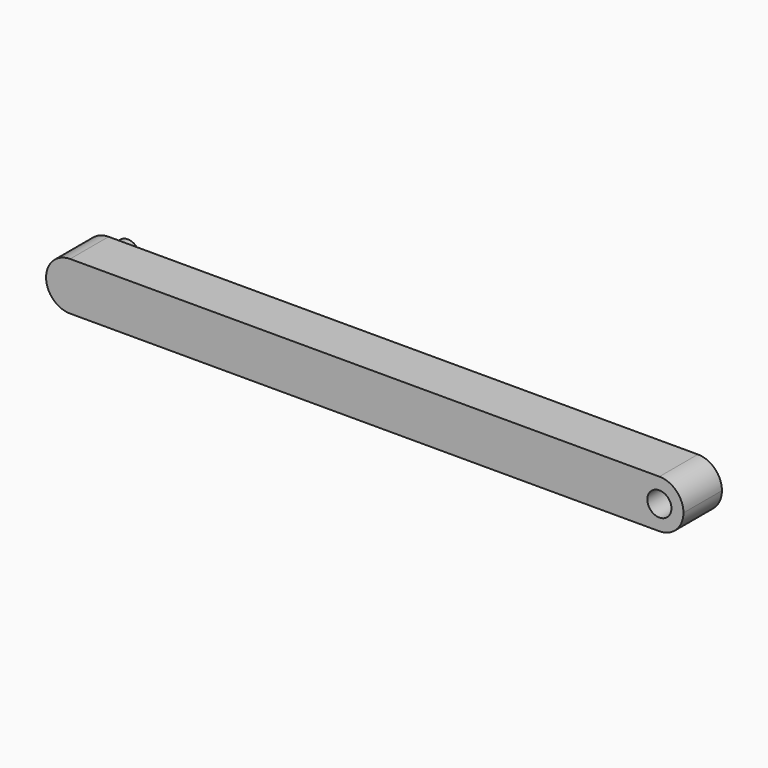
from build123d import *

# Parameters (mm, degrees)
F0_W     = 336.55
F0_H     = 25.4
F1_DEPTH = 25.4
F2_R     = 12.69999
F3_R     = 6.35
F4_DEPTH = 12.7
F5_R     = 6.35
F6_DEPTH = 25.401


# Not quite as in the source:
# - a fillet or chamfer is up to 0.001 mm smaller than in the source, because OpenCascade refuses the exact size


with BuildPart() as f1:
    # F0 (on Front) → F1 (new body)
    with BuildSketch(Plane.XZ):
        with Locations((29.4598335922, -16.8253869212)):
            Rectangle(F0_W, F0_H)
    extrude(amount=F1_DEPTH)

    # F2 (radius 12.7 in the source; OpenCascade refuses exactly that, so slightly less here)
    f2_edges = [f1.edges().sort_by_distance(p)[0] for p in [
        (-138.815166, -12.7, -4.125387),
        (-138.815166, -12.7, -29.525387),
        (197.734834, -12.7, -29.525387),
        (197.734834, -12.7, -4.125387),
    ]]
    fillet(f2_edges, radius=F2_R)

    # F3 (on face) → F4 (join)
    with BuildSketch(Plane(origin=(0, 0, 0), x_dir=(-1, 0, 0), z_dir=(0, 1, 0))):
        with Locations((126.1151664078, -16.8253869212)):
            Circle(F3_R)
    extrude(amount=F4_DEPTH)

    # F5 (on face) → F6 (cut, through all)
    with BuildSketch(Plane(origin=(0, 0, 0), x_dir=(-1, 0, 0), z_dir=(0, 1, 0))):
        with Locations((-185.0348335922, -16.8253869212)):
            Circle(F5_R)
    extrude(amount=-F6_DEPTH, mode=Mode.SUBTRACT)


solid = f1.part
